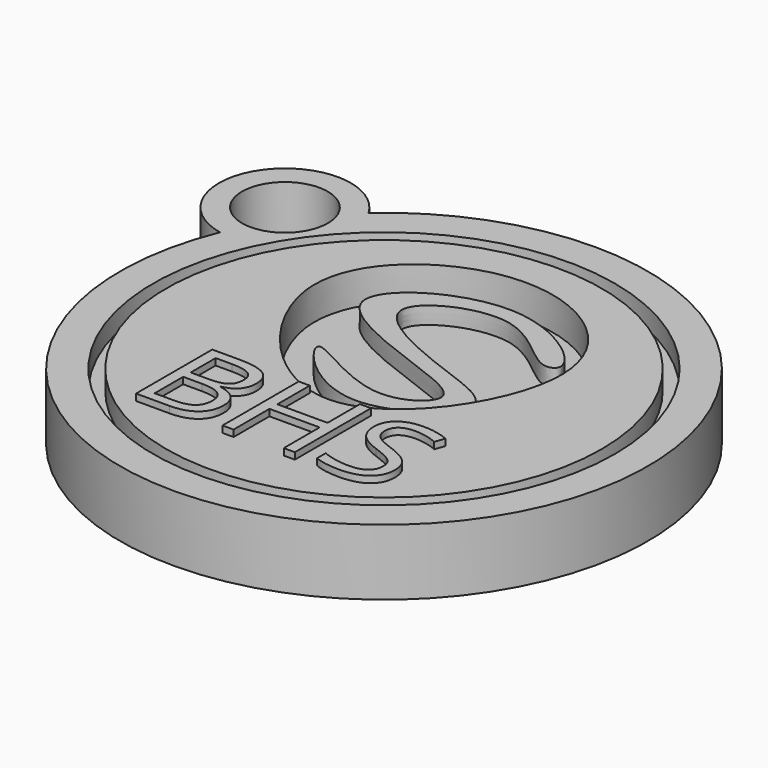
from build123d import *

# Parameters (mm, degrees)
F0_R          = 12.7
F1_DEPTH      = 3.175
F2_R          = 11.1125
F2_R_2        = 10.4775
F3_DEPTH      = 0.9525
F5_DEPTH      = 3.175
F7_DEPTH      = 3.175
F9_DEPTH      = 0.762
F10_DEPTH     = 1.5875
F11_TEXT_SIZE = 6.4215499959
F12_DEPTH     = 0.3175


# Not quite as in the source:
# - Text() gives the source's letters only with a copy of the font that has no kerning and outlines rounded to 1/6400 em; it was checked with that copy


with BuildPart() as f1:
    # F0 (on Top) → F1 (new body)
    with BuildSketch(Plane.XY):
        Circle(F0_R)
    extrude(amount=F1_DEPTH)

    # F2 (on face) → F3 (cut)
    with BuildSketch(Plane.XY.offset(3.175)):
        Circle(F2_R)
        Circle(F2_R_2, mode=Mode.SUBTRACT)
    extrude(amount=-F3_DEPTH, mode=Mode.SUBTRACT)

    # F4 (on face) → F5 (join)
    with BuildSketch(Plane.XY.offset(3.175)):
        with BuildLine():
            ThreePointArc((-11.7495023087, 4.8207048755), (-10.3372093023, 7.3778115888), (-8.3780058038, 9.5445805959))
            ThreePointArc((-8.3780058038, 9.5445805959), (-13.6968023256, 9.7756003552), (-11.7495023087, 4.8207048755))
        make_face()
    extrude(amount=-F5_DEPTH)

    # F6 (on face) → F7 (cut, through all)
    with BuildSketch(Plane.XY.offset(3.175)):
        with BuildLine():
            ThreePointArc((-11.2606028671, 5.8727185417), (-10.3372093023, 7.3778115888), (-9.2139830578, 8.7402812433))
            ThreePointArc((-9.2139830578, 8.7402812433), (-12.7922965116, 9.1300418411), (-11.2606028671, 5.8727185417))
        make_face()
        with BuildLine():
            ThreePointArc((-11.2606028671, 5.8727185417), (-9.7065453829, 6.4204007296), (-9.04875, 7.931147458))
            ThreePointArc((-9.04875, 7.931147458), (-9.090480168, 8.3440637467), (-9.2139830578, 8.7402812433))
            ThreePointArc((-9.2139830578, 8.7402812433), (-10.3372093023, 7.3778115888), (-11.2606028671, 5.8727185417))
        make_face()
    extrude(amount=-F7_DEPTH, mode=Mode.SUBTRACT)

    # F8 (on face) → F9 (cut)
    with BuildSketch(Plane.XY.offset(3.175)):
        with BuildLine():
            add(Edge.make_bspline(
                [(3.556300886, 5.1342109218), (2.7939876064, 5.3393883791), (0.7372922471, 8.2209550976), (-5.4456273068, 5.307801787), (0.3935277103, 2.5296153354), (5.2130663592, 1.1945089003), (-0.1600592941, -2.8789581996), (-3.78085818, 0.1698889621), (-4.2543878059, 1.6422689928), (-0.0549431212, -1.4866214959), (3.1622969891, 0.7785730408), (-0.0329872355, 2.1370393063), (-7.7833970694, 4.7212475559), (0.059091823, 9.4713465914), (4.9007863041, 5.5257089068), (3.8792130997, 5.0472987445), (3.556300886, 5.1342109218)],
                knots=[0, 0, 0, 0, 0.0746569318, 0.1519251632, 0.2352900108, 0.308739673, 0.3882197263, 0.468075104, 0.4967036746, 0.5757141921, 0.6363091973, 0.6989112495, 0.7918952009, 0.8839348496, 0.9683756852, 1, 1, 1, 1], degree=3))
        make_face()
    extrude(amount=-F9_DEPTH, mode=Mode.SUBTRACT)

    # F8 (on face) → F10 (cut)
    with BuildSketch(Plane.XY.offset(3.175)):
        with BuildLine():
            add(Edge.make_bspline(
                [(5.5002495646, 3.3243272919), (5.2676864775, 0.5419120178), (0.2191834939, -7.0069378403), (-8.6962215365, 3.590818838), (-2.9958581648, 9.2156608781), (3.1871096131, 8.8136760712), (5.6854512798, 5.5401048998), (5.5002495646, 3.3243272919)],
                knots=[0, 0, 0, 0, 0.2232520564, 0.4540823142, 0.6422037573, 0.8222131282, 1, 1, 1, 1], degree=3))
        make_face()
        with BuildLine():
            add(Edge.make_bspline(
                [(3.556300886, 5.1342109218), (2.7939876064, 5.3393883791), (0.7372922471, 8.2209550976), (-5.4456273068, 5.307801787), (0.3935277103, 2.5296153354), (5.2130663592, 1.1945089003), (-0.1600592941, -2.8789581996), (-3.78085818, 0.1698889621), (-4.2543878059, 1.6422689928), (-0.0549431212, -1.4866214959), (3.1622969891, 0.7785730408), (-0.0329872355, 2.1370393063), (-7.7833970694, 4.7212475559), (0.059091823, 9.4713465914), (4.9007863041, 5.5257089068), (3.8792130997, 5.0472987445), (3.556300886, 5.1342109218)],
                knots=[0, 0, 0, 0, 0.0746569318, 0.1519251632, 0.2352900108, 0.308739673, 0.3882197263, 0.468075104, 0.4967036746, 0.5757141921, 0.6363091973, 0.6989112495, 0.7918952009, 0.8839348496, 0.9683756852, 1, 1, 1, 1], degree=3))
        make_face(mode=Mode.SUBTRACT)
    extrude(amount=-F10_DEPTH, mode=Mode.SUBTRACT)

    # F11 (on face) → F12 (join)
    with BuildSketch(Plane.XY.offset(3.175)):
        with Locations((-6.266028082, -7.8716650605)):
            Text('BHS', F11_TEXT_SIZE, font='Open Sans', text_align=(TextAlign.LEFT, TextAlign.BOTTOM))
    extrude(amount=F12_DEPTH)


solid = f1.part
